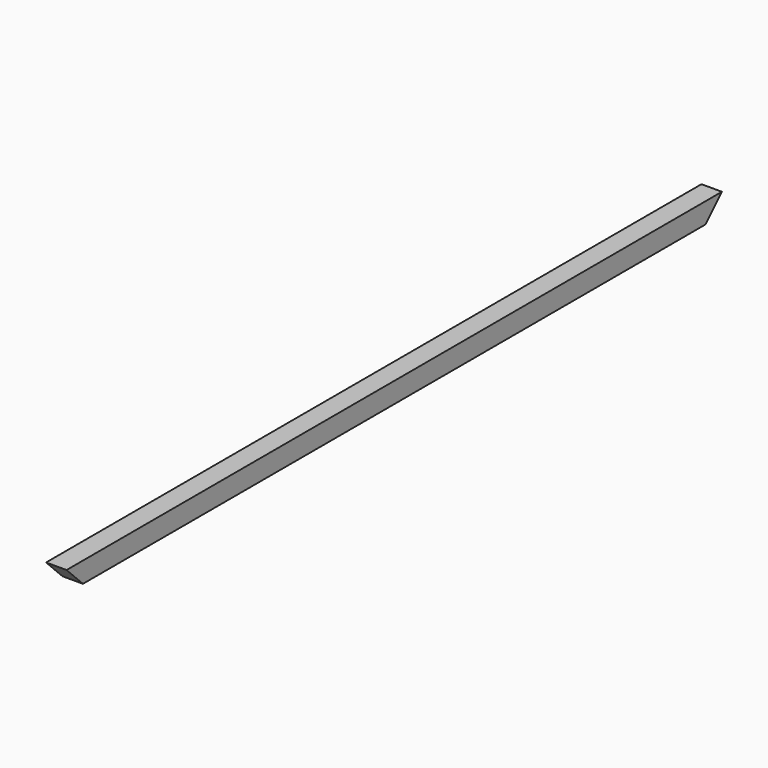
from build123d import *

# Parameters (mm, degrees)
F0_W     = 3.81
F0_H     = 152.4
F1_DEPTH = 3.81
F2_SIZE  = 3.80999
F3_SIZE  = 3.80999


# Not quite as in the source:
# - a fillet or chamfer is up to 0.001 mm smaller than in the source, because OpenCascade refuses the exact size


with BuildPart() as f1:
    # F0 (on Top) → F1 (new body)
    with BuildSketch(Plane.XY):
        with Locations((-48.8890688866, 24.7670258315)):
            Rectangle(F0_W, F0_H)
    extrude(amount=F1_DEPTH)

    # F2 (size 3.81 in the source; OpenCascade refuses exactly that, so slightly less here)
    f2_edges = [f1.edges().sort_by_distance(p)[0] for p in [
        (-48.889069, -51.432974, 0),
    ]]
    chamfer(f2_edges, length=F2_SIZE)

    # F3 (size 3.81 in the source; OpenCascade refuses exactly that, so slightly less here)
    f3_edges = [f1.edges().sort_by_distance(p)[0] for p in [
        (-48.889069, 100.967026, 0),
    ]]
    chamfer(f3_edges, length=F3_SIZE)


solid = f1.part
